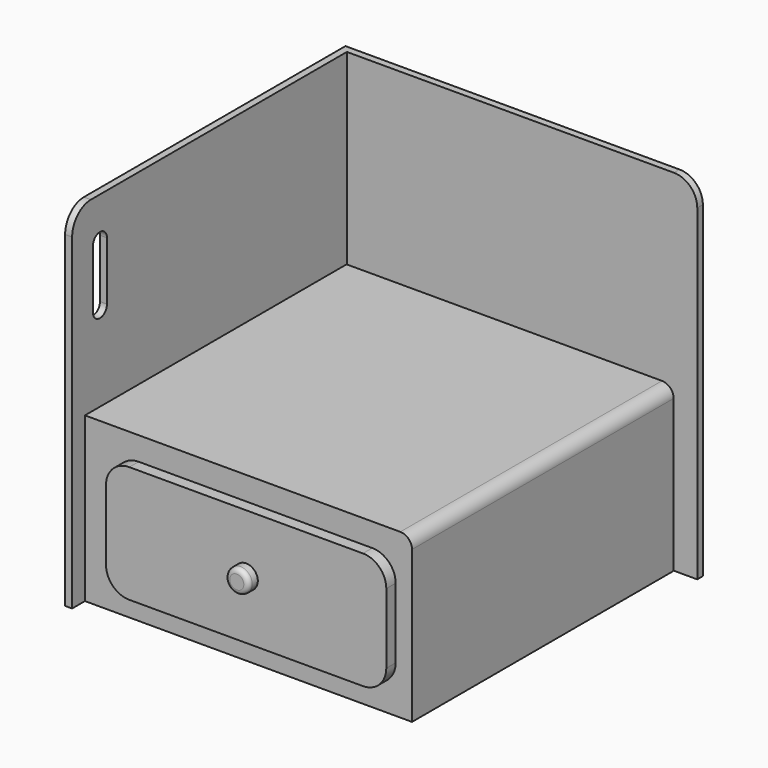
from build123d import *

# Parameters (mm, degrees)
F0_W      = 38.1
F0_H      = 38.1
F2_DEPTH  = 0.762
F1_W      = 38.1
F1_H      = 38.1
F3_DEPTH  = 0.762
F4_W      = 35.56
F4_H      = 35.56
F5_DEPTH  = 17.78
F6_W      = 30.48
F6_H      = 12.7
F7_DEPTH  = 1.27
F8_R      = 1.27
F9_DEPTH  = 1.27
F10_R     = 2.54
F11_R     = 1.27
F13_DEPTH = 25.4
F14_R     = 0.508
F15_R     = 2.54
F16_R     = 2.54


with BuildPart() as f2:
    # F0 (on Right) → F2 (new body)
    with BuildSketch(Plane.YZ):
        with Locations((-19.05, 19.05)):
            Rectangle(F0_W, F0_H)
    extrude(amount=-F2_DEPTH)

    # F1 (on Front) → F3 (join)
    with BuildSketch(Plane.XZ):
        with Locations((19.05, 19.05)):
            Rectangle(F1_W, F1_H)
    extrude(amount=F3_DEPTH)

    # F10
    f10_edges = [f2.edges().sort_by_distance(p)[0] for p in [
        (-0.381, -38.1, 38.1),
    ]]
    fillet(f10_edges, radius=F10_R)

    # F12 (on face) → F13 (cut)
    with BuildSketch(Plane(origin=(-0.762, 0, 0), x_dir=(0, -1, 0), z_dir=(-1, 0, 0))):
        with BuildLine():
            ThreePointArc((35.2714537645, 33.5571871057), (34.3189537645, 34.5096871057), (33.3664537645, 33.5571871057))
            Line((33.3664537645, 33.5571871057), (33.3664537645, 27.2071871057))
            ThreePointArc((33.3664537645, 27.2071871057), (34.3189537645, 26.2546871057), (35.2714537645, 27.2071871057))
            Line((35.2714537645, 27.2071871057), (35.2714537645, 33.5571871057))
        make_face()
    extrude(amount=-F13_DEPTH, mode=Mode.SUBTRACT)

    # F16
    f16_edges = [f2.edges().sort_by_distance(p)[0] for p in [
        (38.1, -0.381, 38.1),
    ]]
    fillet(f16_edges, radius=F16_R)


with BuildPart() as f5:
    # F4 (on Top) → F5 (new body)
    with BuildSketch(Plane.XY):
        with Locations((17.78, -18.5785688174)):
            Rectangle(F4_W, F4_H)
    extrude(amount=F5_DEPTH)

    # F11
    f11_edges = [f5.edges().sort_by_distance(p)[0] for p in [
        (35.56, -18.578569, 17.78),
    ]]
    fillet(f11_edges, radius=F11_R)


with BuildPart() as f7:
    # F6 (on face) → F7 (new body)
    with BuildSketch(Plane.XZ.offset(36.3585688174)):
        with Locations((18.542, 8.89)):
            Rectangle(F6_W, F6_H)
    extrude(amount=F7_DEPTH)

    # F15
    f15_edges = [f7.edges().sort_by_distance(p)[0] for p in [
        (3.302, -36.993569, 15.24),
        (3.302, -36.993569, 2.54),
        (33.782, -36.993569, 2.54),
        (33.782, -36.993569, 15.24),
    ]]
    fillet(f15_edges, radius=F15_R)


with BuildPart() as f9:
    # F8 (on face) → F9 (new body)
    with BuildSketch(Plane.XZ.offset(37.6285688174)):
        with Locations((18.542, 8.89)):
            Circle(F8_R)
    extrude(amount=F9_DEPTH)

    # F14
    f14_edges = [f9.edges().sort_by_distance(p)[0] for p in [
        (17.272, -38.898569, 8.89),
    ]]
    fillet(f14_edges, radius=F14_R)


solid = Compound([f2.part, f5.part, f7.part, f9.part])
